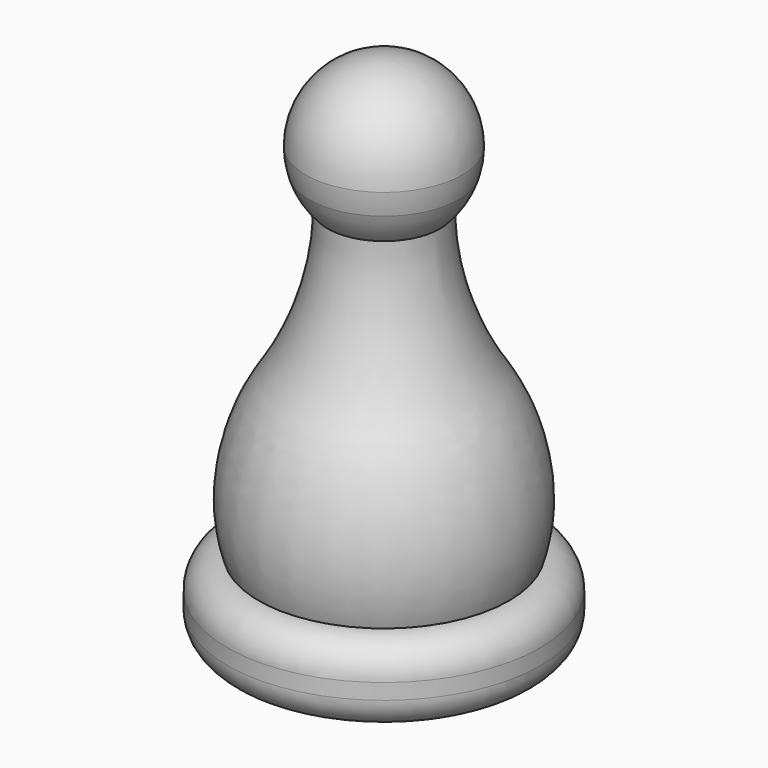
from build123d import *

# Parameters (mm, degrees)
F2_R = 1.99999
F3_R = 2


# Not quite as in the source:
# - a fillet or chamfer is up to 0.001 mm smaller than in the source, because OpenCascade refuses the exact size
# - after a boolean that leaves OpenCascade's solid faulty, fix() repairs it


with BuildPart() as f1:
    # F0 (on Front) → F1 (revolve)
    with BuildSketch(Plane.XZ):
        with BuildLine():
            Line((0, 22.9767435235), (0, 0))
            Line((0, 0), (10, 0))
            Line((10, 0), (10, 5))
            Line((10, 5), (8, 5))
            add(Edge.make_bspline(
                [(8, 5), (9.090302038, 8.3032843893), (7.5695253902, 13.5642188714), (5.5203949762, 15.97344633), (3.4543829705, 21.1989798105), (3.5896653484, 24.4961828379)],
                knots=[0, 0, 0, 0, 0.3799051131, 0.6150582777, 1, 1, 1, 1], degree=3))
            ThreePointArc((3.5896653484, 24.4961828379), (1.9489993037, 23.3722455363), (0, 22.9767435235))
        make_face()
        with BuildLine():
            Line((0, 26.5213213809), (0, 22.9767435235))
            ThreePointArc((0, 22.9767435235), (1.9489993037, 23.3722455363), (3.5896653484, 24.4961828379))
            ThreePointArc((3.5896653484, 24.4961828379), (4.3072863776, 25.4375932599), (4.783486844, 26.5213213809))
            Line((4.783486844, 26.5213213809), (0, 26.5213213809))
        make_face()
        with BuildLine():
            ThreePointArc((-5, 27.9767435235), (-4.9455755085, 27.2410242224), (-4.783486844, 26.5213213809))
            Line((-4.783486844, 26.5213213809), (0, 26.5213213809))
            Line((0, 26.5213213809), (0, 27.9767435235))
            Line((0, 27.9767435235), (-5, 27.9767435235))
        make_face()
        with BuildLine():
            Line((0, 32.9767435235), (0, 27.9767435235))
            Line((0, 27.9767435235), (5, 27.9767435235))
            ThreePointArc((5, 27.9767435235), (3.5355339059, 31.5122774294), (0, 32.9767435235))
        make_face()
    revolve(axis=Axis((0, 0, 30.4767435235), (0, 0, 1)))

    add(f1.part.fix(), mode=Mode.REPLACE)

    # F2 (radius 2 in the source; OpenCascade refuses exactly that, so slightly less here)
    f2_edges = [f1.edges().sort_by_distance(p)[0] for p in [
        (-10, 0, 5),
    ]]
    fillet(f2_edges, radius=F2_R)

    # F3
    f3_edges = [f1.edges().sort_by_distance(p)[0] for p in [
        (-10, 0, 0),
    ]]
    fillet(f3_edges, radius=F3_R)


solid = f1.part
